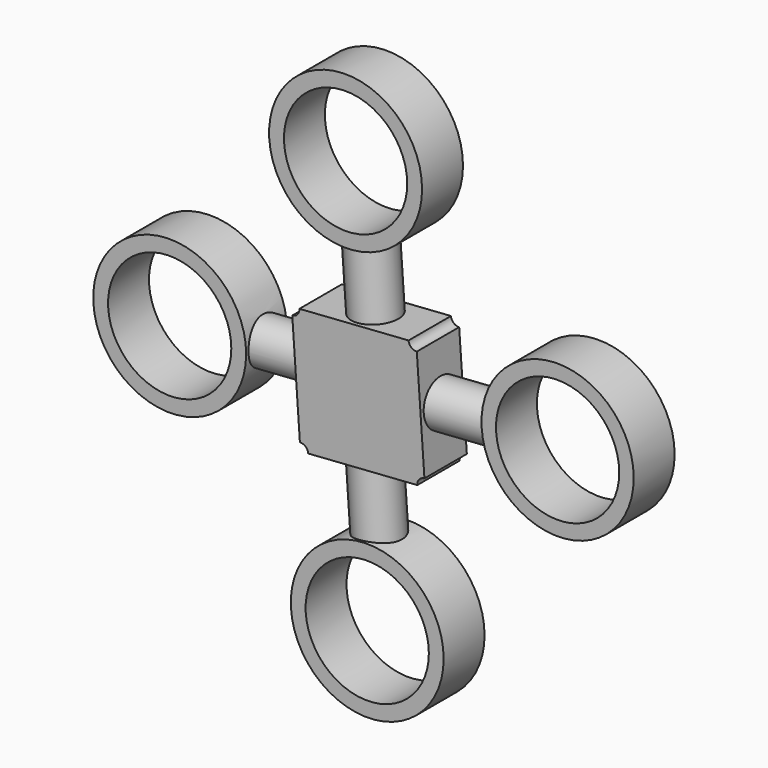
from build123d import *

# Parameters (mm, degrees)
F1_DEPTH  = 21.844
F5_R      = 9.3558336569
F6_DEPTH  = 58.42
F3_R      = 9.4583600755
F7_DEPTH  = 55.626
F4_R      = 9.3478497533
F8_DEPTH  = 52.832
F2_R      = 9.4635805484
F9_DEPTH  = 58.42
F12_R     = 31.3770390823
F10_R     = 31.5053231156
F11_R     = 31.5183409025
F13_R     = 31.5308798418
F14_DEPTH = 21.082
F21_D     = 6.35
F23_D     = 50.8
F25_D     = 50.8
F27_D     = 50.8
F29_D     = 50.8


# Not quite as in the source:
# - the program builds the solid bodies; features that only make, move or delete a surface that nothing else refers to are left out


with BuildPart() as f1:
    # F0 (on Front) → F1 (new body)
    with BuildSketch(Plane.XZ):
        Polygon((23.8739177585, 27.4659190327), (-27.4659190327, 23.8739177585), (-23.8739177585, -27.4659190327), (27.4659190327, -23.8739177585), align=None)
    extrude(amount=F1_DEPTH)

    # F5 (on face) → F6 (join)
    with BuildSketch(Plane(origin=(1.7960006371, 0, -25.6699183956), x_dir=(0.9975613857, 0, 0.0697945687), z_dir=(0.0697945687, 0, -0.9975613857))):
        with Locations((-3.9608110674, 10.7757570222)):
            Circle(F5_R)
    extrude(amount=F6_DEPTH)

    # F3 (on face) → F7 (join)
    with BuildSketch(Plane(origin=(25.6699183956, 0, 1.7960006371), x_dir=(0, 1, 0), z_dir=(0.9975613857, 0, 0.0697945687))):
        with Locations((-10.7757570222, 0)):
            Circle(F3_R)
    extrude(amount=F7_DEPTH)

    # F4 (on face) → F8 (join)
    with BuildSketch(Plane(origin=(-25.6699183956, 0, -1.7960006371), x_dir=(0, -1, 0), z_dir=(-0.9975613857, 0, -0.0697945687))):
        with Locations((10.5063626543, 3.6907584872)):
            Circle(F4_R)
    extrude(amount=F8_DEPTH)

    # F2 (on face) → F9 (join)
    with BuildSketch(Plane(origin=(-1.7960006371, 0, 25.6699183956), x_dir=(0.9975613857, 0, 0.0697945687), z_dir=(-0.0697945687, 0, 0.9975613857))):
        with Locations((0, -10.7757570222)):
            Circle(F2_R)
    extrude(amount=F9_DEPTH)

    # F12 (on Front) + F10 (on Front) + F11 (on Front) + F13 (on Front) → F14 (join)
    with BuildSketch(Plane.XZ):
        with Locations((81.530354917, 6.9857356139)):
            Circle(F12_R)
    with BuildSketch(Plane.XZ):
        with Locations((3.051524749, -84.1294080019)):
            Circle(F10_R)
    with BuildSketch(Plane.XZ):
        with Locations((-78.3801749349, 0)):
            Circle(F11_R)
    with BuildSketch(Plane.XZ):
        with Locations((-5.8717224747, 83.4135636687)):
            Circle(F13_R)
    extrude(amount=F14_DEPTH)

    # F21 (through all)
    with Locations(Plane(origin=(0, 0, 0), x_dir=(-1, 0, 0), z_dir=(0, 1, 0))):
        with Locations((23.8739177585, -27.4659190327), (-27.4659190327, -23.8739177585), (-23.8739177585, 27.4659190327), (27.4659190327, 23.8739177585)):
            Hole(F21_D / 2)

    # F23 (through all)
    with Locations(Plane(origin=(0, 0, 0), x_dir=(-1, 0, 0), z_dir=(0, 1, 0))):
        with Locations((5.8717224747, 83.4135636687)):
            Hole(F23_D / 2)

    # F25 (through all)
    with Locations(Plane(origin=(0, 0, 0), x_dir=(-1, 0, 0), z_dir=(0, 1, 0))):
        with Locations((-81.530354917, 6.9857356139)):
            Hole(F25_D / 2)

    # F27 (through all)
    with Locations(Plane(origin=(0, 0, 0), x_dir=(-1, 0, 0), z_dir=(0, 1, 0))):
        with Locations((78.3801749349, 0)):
            Hole(F27_D / 2)

    # F29 (through all)
    with Locations(Plane(origin=(0, 0, 0), x_dir=(-1, 0, 0), z_dir=(0, 1, 0))):
        with Locations((-3.051524749, -84.1294080019)):
            Hole(F29_D / 2)


solid = f1.part
